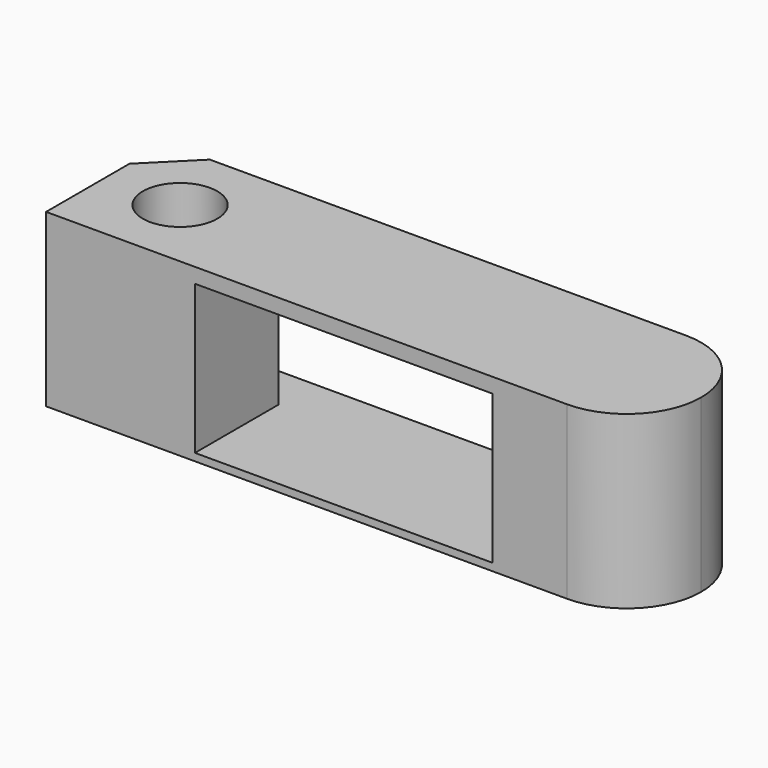
from build123d import *

# Parameters (mm, degrees)
F0_W     = 40
F0_H     = 10
F1_DEPTH = 0.5
F2_W     = 10
F2_H     = 10
F3_DEPTH = 10
F4_W     = 10
F4_H     = 10
F4_W_2   = 30
F5_DEPTH = 1
F6_R     = 4.99999
F7_R     = 2.5
F8_DEPTH = 25
F9_SIZE  = 3


# Not quite as in the source:
# - a fillet or chamfer is up to 0.001 mm smaller than in the source, because OpenCascade refuses the exact size


with BuildPart() as f1:
    # F0 (on Top) → F1 (new body)
    with BuildSketch(Plane.XY):
        Rectangle(F0_W, F0_H)
    extrude(amount=F1_DEPTH)

    # F2 (on face) → F3 (join)
    with BuildSketch(Plane.XY.offset(0.5)):
        with Locations((-15, 0)):
            Rectangle(F2_W, F2_H)
        with Locations((15, 0)):
            Rectangle(F2_W, F2_H)
    extrude(amount=F3_DEPTH)

    # F4 (on face) → F5 (join)
    with BuildSketch(Plane.XY.offset(10.5)):
        with Locations((-15, 0)):
            Rectangle(F4_W, F4_H)
        with Locations((5, 0)):
            Rectangle(F4_W_2, F4_H)
    extrude(amount=F5_DEPTH)

    # F6 (radius 5 in the source; OpenCascade refuses exactly that, so slightly less here)
    f6_edges = [f1.edges().sort_by_distance(p)[0] for p in [
        (20, -5, 5.75),
        (20, 5, 5.75),
    ]]
    fillet(f6_edges, radius=F6_R)

    # F7 (on face) → F8 (cut)
    with BuildSketch(Plane.XY.offset(11.5)):
        with Locations((-15, 0)):
            Circle(F7_R)
    extrude(amount=-F8_DEPTH, mode=Mode.SUBTRACT)

    # F9
    f9_edges = [f1.edges().sort_by_distance(p)[0] for p in [
        (-20, 5, 5.75),
        (-10, 5, 5.5),
    ]]
    chamfer(f9_edges, length=F9_SIZE)


solid = f1.part
